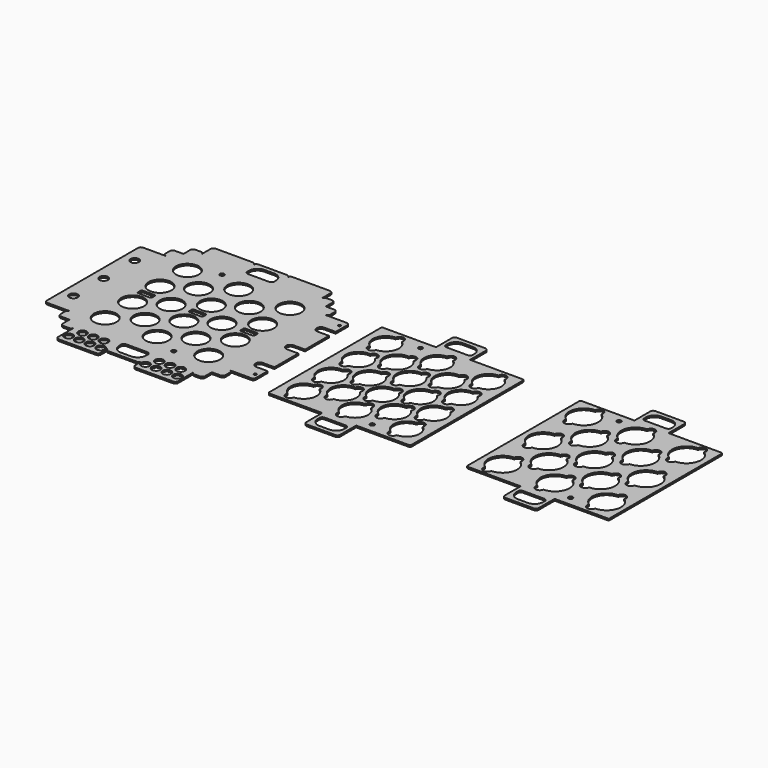
from build123d import *

# Parameters (mm, degrees)
F0_R     = 15
F0_R_2   = 40
F0_R_3   = 7.5
F0_R_4   = 4.25
F1_DEPTH = 6
F2_R     = 7.5
F3_DEPTH = 6
F4_DEPTH = 6


# Not quite as in the source:
# - ends of sketch curves that miss each other by under 0.0002 mm in the source are joined
# - a feature names something its author has since deleted; it is built from what else it names


with BuildPart() as f1:
    # F0 (on Top) → F1 (new body)
    with BuildSketch(Plane.XY):
        with BuildLine():
            Line((-30, 0), (0, 0))
            Line((0, 0), (0, -30))
            ThreePointArc((0, -30), (2.9289321881, -37.0710678119), (10, -40))
            Line((10, -40), (30, -40))
            ThreePointArc((30, -40), (37.0710678119, -37.0710678119), (40, -30))
            Line((40, -30), (40, -70))
            Line((40, -70), (40, -100))
            ThreePointArc((40, -100), (42.9289321881, -107.0710678119), (50, -110))
            Line((50, -110), (181, -110))
            ThreePointArc((181, -110), (188.0710678119, -107.0710678119), (191, -100))
            Line((191, -100), (191, -70))
            ThreePointArc((191, -70), (193.9289321881, -77.0710678119), (201, -80))
            Line((201, -80), (251, -80))
            Line((251, -80), (301, -80))
            ThreePointArc((301, -80), (308.0710678119, -77.0710678119), (311, -70))
            Line((311, -70), (311, -99.9810798484))
            ThreePointArc((311, -99.9810798484), (313.9356373432, -107.0588464633), (321.0189560508, -109.9810618818))
            Line((321.0189560508, -109.9810618818), (452.8887964343, -109.7310882936))
            ThreePointArc((452.8887964343, -109.7310882936), (459.9476069984, -106.795468917), (462.8698403835, -99.7311062602))
            Line((462.8698403835, -99.7311062602), (462.8698403835, -30))
            ThreePointArc((462.8698403835, -30), (465.7987725717, -37.0710678119), (472.8698403835, -40))
            Line((472.8698403835, -40), (492, -40))
            ThreePointArc((492, -40), (499.0710678119, -37.0710678119), (502, -30))
            Line((502, -30), (502, 0))
            Line((502, 0), (532, 0))
            ThreePointArc((532, 0), (539.0710678119, 2.9289321881), (542, 10))
            Line((542, 10), (542, 30))
            ThreePointArc((542, 30), (539.0710678119, 37.0710678119), (532, 40))
            Line((532, 40), (608, 40))
            ThreePointArc((608, 40), (615.0710678119, 42.9289321881), (618, 50))
            Line((618, 50), (618, 101))
            Line((618, 101), (578, 101))
            ThreePointArc((578, 101), (563, 116), (578, 131))
            Line((578, 131), (618, 131))
            Line((618, 131), (618, 236))
            Line((618, 236), (578, 236))
            ThreePointArc((578, 236), (563, 251), (578, 266))
            Line((578, 266), (618, 266))
            Line((618, 266), (618, 371))
            Line((618, 371), (578, 371))
            ThreePointArc((578, 371), (563, 386), (578, 401))
            Line((578, 401), (618, 401))
            Line((618, 401), (618, 452))
            ThreePointArc((618, 452), (615.0710678119, 459.0710678119), (608, 462))
            Line((608, 462), (532, 462))
            ThreePointArc((532, 462), (539.0710678119, 464.9289321881), (542, 472))
            Line((542, 472), (542, 492))
            ThreePointArc((542, 492), (539.0710678119, 499.0710678119), (532, 502))
            Line((532, 502), (502, 502))
            Line((502, 502), (502, 532))
            ThreePointArc((502, 532), (499.0710678119, 539.0710678119), (492, 542))
            Line((492, 542), (472.8698403835, 542))
            ThreePointArc((472.8698403835, 542), (465.7987725717, 539.0710678119), (462.8698403835, 532))
            Line((462.8698403835, 532), (462.8698403835, 572))
            ThreePointArc((462.8698403835, 572), (459.9409081954, 579.0710678119), (452.8698403835, 582))
            Line((452.8698403835, 582), (321, 582))
            ThreePointArc((321, 582), (313.9289321881, 579.0710678119), (311, 572))
            ThreePointArc((311, 572), (308.0710678119, 579.0710678119), (301, 582))
            Line((301, 582), (251, 582))
            Line((251, 582), (201, 582))
            ThreePointArc((201, 582), (193.9289321881, 579.0710678119), (191, 572))
            ThreePointArc((191, 572), (188.0710678119, 579.0710678119), (181, 582))
            Line((181, 582), (50, 582))
            ThreePointArc((50, 582), (42.9289321881, 579.0710678119), (40, 572))
            Line((40, 572), (40, 532))
            ThreePointArc((40, 532), (37.0710678119, 539.0710678119), (30, 542))
            Line((30, 542), (10, 542))
            ThreePointArc((10, 542), (2.9289321881, 539.0710678119), (0, 532))
            Line((0, 532), (0, 502))
            Line((0, 502), (-30, 502))
            ThreePointArc((-30, 502), (-37.0710678119, 499.0710678119), (-40, 492))
            Line((-40, 492), (-40, 472))
            ThreePointArc((-40, 472), (-37.0710678119, 464.9289321881), (-30, 462))
            Line((-30, 462), (-110, 462))
            ThreePointArc((-110, 462), (-117.0710678119, 459.0710678119), (-120, 452))
            Line((-120, 452), (-120, 251))
            Line((-120, 251), (-120, 50))
            ThreePointArc((-120, 50), (-117.0710678119, 42.9289321881), (-110, 40))
            Line((-110, 40), (-30, 40))
            ThreePointArc((-30, 40), (-37.0710678119, 37.0710678119), (-40, 30))
            Line((-40, 30), (-40, 10))
            ThreePointArc((-40, 10), (-37.0710678119, 2.9289321881), (-30, 0))
        make_face()
        with Locations((58.8749991059, -77.75)):
            Circle(F0_R, mode=Mode.SUBTRACT)
        with Locations((96.6249991059, -77.75)):
            Circle(F0_R, mode=Mode.SUBTRACT)
        with Locations((134.3749991059, -77.75)):
            Circle(F0_R, mode=Mode.SUBTRACT)
        with Locations((77.7499991059, -40)):
            Circle(F0_R, mode=Mode.SUBTRACT)
        with Locations((115.4999991059, -40)):
            Circle(F0_R, mode=Mode.SUBTRACT)
        with Locations((153.2499991059, -40)):
            Circle(F0_R, mode=Mode.SUBTRACT)
        with Locations((172.1249991059, -77.75)):
            Circle(F0_R, mode=Mode.SUBTRACT)
        with Locations((-80, 117.4095802605)):
            Circle(F0_R, mode=Mode.SUBTRACT)
        with Locations((70.0655404942, 69.6284726141)):
            Circle(F0_R_2, mode=Mode.SUBTRACT)
        with Locations((162.0928294033, 130.3333938122)):
            Circle(F0_R_2, mode=Mode.SUBTRACT)
        with Locations((70, 190.6667947769)):
            Circle(F0_R_2, mode=Mode.SUBTRACT)
        with Locations((329.8749991059, -77.75)):
            Circle(F0_R, mode=Mode.SUBTRACT)
        with BuildLine():
            Line((298.4369397163, -27.4369397163), (298.4369397163, -35))
            ThreePointArc((298.4369397163, -35), (289.6501431519, -56.2132034356), (268.4369397163, -65))
            Line((268.4369397163, -65), (233.5630602837, -65))
            ThreePointArc((233.5630602837, -65), (212.3498568481, -56.2132034356), (203.5630602837, -35))
            Line((203.5630602837, -35), (203.5630602837, -27.4369397163))
            ThreePointArc((203.5630602837, -27.4369397163), (206.4919924718, -20.3658719045), (213.5630602837, -17.4369397163))
            Line((213.5630602837, -17.4369397163), (288.4369397163, -17.4369397163))
            ThreePointArc((288.4369397163, -17.4369397163), (295.5080075282, -20.3658719045), (298.4369397163, -27.4369397163))
        make_face(mode=Mode.SUBTRACT)
        with Locations((367.6249991059, -77.75)):
            Circle(F0_R, mode=Mode.SUBTRACT)
        with Locations((405.3749991059, -77.75)):
            Circle(F0_R, mode=Mode.SUBTRACT)
        with Locations((348.7499991059, -40)):
            Circle(F0_R, mode=Mode.SUBTRACT)
        with Locations((386.4999991059, -40)):
            Circle(F0_R, mode=Mode.SUBTRACT)
        with Locations((424.2499991059, -40)):
            Circle(F0_R, mode=Mode.SUBTRACT)
        with Locations((341.500023365, 32.5)):
            Circle(F0_R_3, mode=Mode.SUBTRACT)
        with Locations((443.1249991059, -77.75)):
            Circle(F0_R, mode=Mode.SUBTRACT)
        with Locations((250.9999752045, 72.1276074222)):
            Circle(F0_R_2, mode=Mode.SUBTRACT)
        with Locations((432.5207205657, 72.8690030603)):
            Circle(F0_R_2, mode=Mode.SUBTRACT)
        with Locations((341.4999717873, 130.3333938122)):
            Circle(F0_R_2, mode=Mode.SUBTRACT)
        with Locations((250.999969244, 190.6667947769)):
            Circle(F0_R_2, mode=Mode.SUBTRACT)
        with BuildLine():
            ThreePointArc((431.9999940395, 230.6666), (432.2603582464, 230.665752622), (432.520711422, 230.663210524))
            ThreePointArc((432.520711422, 230.663210524), (460.4677713966, 218.7661667645), (471.9999940395, 190.6666))
            ThreePointArc((471.9999940395, 190.6666), (403.7157227921, 162.3823287525), (431.9999940395, 230.6666))
        make_face(mode=Mode.SUBTRACT)
        with Locations((603, 65)):
            Circle(F0_R_4, mode=Mode.SUBTRACT)
        with Locations((-80, 251)):
            Circle(F0_R, mode=Mode.SUBTRACT)
        with Locations((-80, 387.4095802605)):
            Circle(F0_R, mode=Mode.SUBTRACT)
        with BuildLine():
            Line((95, 256), (95, 246))
            ThreePointArc((95, 246), (93.5355339059, 242.4644660941), (90, 241))
            Line((90, 241), (50, 241))
            ThreePointArc((50, 241), (46.4644660941, 242.4644660941), (45, 246))
            Line((45, 246), (45, 256))
            ThreePointArc((45, 256), (46.4644660941, 259.5355339059), (50, 261))
            Line((50, 261), (90, 261))
            ThreePointArc((90, 261), (93.5355339059, 259.5355339059), (95, 256))
        make_face(mode=Mode.SUBTRACT)
        with Locations((70, 311.3332052231)):
            Circle(F0_R_2, mode=Mode.SUBTRACT)
        with Locations((162.1251841753, 245.0216537661)):
            Circle(F0_R_2, mode=Mode.SUBTRACT)
        with Locations((162.1251583099, 365.6882350202)):
            Circle(F0_R_2, mode=Mode.SUBTRACT)
        with Locations((70, 431.9998052231)):
            Circle(F0_R_2, mode=Mode.SUBTRACT)
        with Locations((160.5000174046, 471.9999026115)):
            Circle(F0_R_3, mode=Mode.SUBTRACT)
        with BuildLine():
            ThreePointArc((231.0000407696, 241), (227.4645068636, 242.4644660941), (226.0000407696, 246))
            Line((226.0000407696, 246), (226.0000407696, 256))
            ThreePointArc((226.0000407696, 256), (227.4645068636, 259.5355339059), (231.0000407696, 261))
            Line((231.0000407696, 261), (271.0000407696, 261))
            ThreePointArc((271.0000407696, 261), (274.5355746755, 259.5355339059), (276.0000407696, 256))
            Line((276.0000407696, 256), (276.0000407696, 246))
            ThreePointArc((276.0000407696, 246), (274.5355746755, 242.4644660941), (271.0000407696, 241))
            Line((271.0000407696, 241), (231.0000407696, 241))
        make_face(mode=Mode.SUBTRACT)
        with Locations((250.999969244, 311.3333880901)):
            Circle(F0_R_2, mode=Mode.SUBTRACT)
        with Locations((341.5323265593, 245.0216537661)):
            Circle(F0_R_2, mode=Mode.SUBTRACT)
        with BuildLine():
            Line((457.5207149068, 255.9999994954), (457.5207138976, 245.9999994954))
            ThreePointArc((457.5207138976, 245.9999994954), (456.0562476252, 242.4644659157), (452.5207138976, 241))
            Line((452.5207138976, 241), (412.520711422, 241))
            ThreePointArc((412.520711422, 241), (408.985177516, 242.4644660941), (407.520711422, 246))
            Line((407.520711422, 246), (407.520711422, 256))
            ThreePointArc((407.520711422, 256), (408.985177516, 259.5355339059), (412.520711422, 261))
            Line((412.520711422, 261), (452.5207149068, 261))
            ThreePointArc((452.5207149068, 261), (456.0562489911, 259.5355337275), (457.5207149068, 255.9999994954))
        make_face(mode=Mode.SUBTRACT)
        with BuildLine():
            ThreePointArc((432.5207173824, 271.3365946991), (432.2603642069, 271.3340526011), (432, 271.3332052231))
            ThreePointArc((432, 271.3332052231), (403.7157287525, 339.6174764705), (472, 311.3332052231))
            ThreePointArc((472, 311.3332052231), (460.467777357, 283.2336384586), (432.5207173824, 271.3365946991))
        make_face(mode=Mode.SUBTRACT)
        with Locations((341.5323006939, 365.6882350202)):
            Circle(F0_R_2, mode=Mode.SUBTRACT)
        with Locations((251.0000348091, 432)):
            Circle(F0_R_2, mode=Mode.SUBTRACT)
        with Locations((432.0000112057, 431.9922370985)):
            Circle(F0_R_2, mode=Mode.SUBTRACT)
        with BuildLine():
            Line((288.4369397163, 519.4369397163), (213.5630602837, 519.4369397163))
            ThreePointArc((213.5630602837, 519.4369397163), (206.4919924718, 522.3658719045), (203.5630602837, 529.4369397163))
            Line((203.5630602837, 529.4369397163), (203.5630602837, 537))
            ThreePointArc((203.5630602837, 537), (212.3498568481, 558.2132034356), (233.5630602837, 567))
            Line((233.5630602837, 567), (268.4369397163, 567))
            ThreePointArc((268.4369397163, 567), (289.6501431519, 558.2132034356), (298.4369397163, 537))
            Line((298.4369397163, 537), (298.4369397163, 529.4369397163))
            ThreePointArc((298.4369397163, 529.4369397163), (295.5080075282, 522.3658719045), (288.4369397163, 519.4369397163))
        make_face(mode=Mode.SUBTRACT)
        with Locations((603, 437)):
            Circle(F0_R_4, mode=Mode.SUBTRACT)
    extrude(amount=F1_DEPTH)


with BuildPart() as f3:
    # F2 (on Top) → F3 (new body)
    with BuildSketch(Plane.XY):
        with BuildLine():
            ThreePointArc((700, 5), (701.4644660941, 1.4644660941), (705, 0))
            Line((705, 0), (891.0000348091, 0))
            Line((891.0000348091, 0), (891.0000348091, -70))
            ThreePointArc((891.0000348091, -70), (893.9289669972, -77.0710678119), (901.0000348091, -80))
            Line((901.0000348091, -80), (1001.0000348091, -80))
            ThreePointArc((1001.0000348091, -80), (1008.071102621, -77.0710678119), (1011.0000348091, -70))
            Line((1011.0000348091, -70), (1011.0000348091, 0))
            Line((1011.0000348091, 0), (1197, 0))
            ThreePointArc((1197, 0), (1200.5355339059, 1.4644660941), (1202, 5))
            Line((1202, 5), (1202, 497))
            ThreePointArc((1202, 497), (1200.5355339059, 500.5355339059), (1197, 502))
            Line((1197, 502), (1011.0000348091, 502))
            Line((1011.0000348091, 502), (1011.0000348091, 572))
            ThreePointArc((1011.0000348091, 572), (1008.071102621, 579.0710678119), (1001.0000348091, 582))
            Line((1001.0000348091, 582), (951.0000348091, 582))
            Line((951.0000348091, 582), (901.0000348091, 582))
            ThreePointArc((901.0000348091, 582), (893.9289669972, 579.0710678119), (891.0000348091, 572))
            Line((891.0000348091, 572), (891.0000348091, 502))
            Line((891.0000348091, 502), (705, 502))
            ThreePointArc((705, 502), (701.4644660941, 500.5355339059), (700, 497))
            Line((700, 497), (700, 5))
        make_face()
        with BuildLine():
            ThreePointArc((903.5630950928, -27.4369397163), (906.4920272809, -20.3658719045), (913.5630950928, -17.4369397163))
            Line((913.5630950928, -17.4369397163), (988.4369745255, -17.4369397163))
            ThreePointArc((988.4369745255, -17.4369397163), (995.5080423373, -20.3658719045), (998.4369745255, -27.4369397163))
            Line((998.4369745255, -27.4369397163), (998.4369745255, -35))
            ThreePointArc((998.4369745255, -35), (989.650177961, -56.2132034356), (968.4369745255, -65))
            Line((968.4369745255, -65), (933.5630950928, -65))
            ThreePointArc((933.5630950928, -65), (912.3498916572, -56.2132034356), (903.5630950928, -35))
            Line((903.5630950928, -35), (903.5630950928, -27.4369397163))
        make_face(mode=Mode.SUBTRACT)
        with BuildLine():
            ThreePointArc((743.4629290669, 32.1011350421), (725.9747079734, 82.7432920036), (768.2980336481, 115.5945026749))
            ThreePointArc((768.2980336481, 115.5945026749), (787.4569314238, 128.0967505221), (796.6681519216, 107.1558101861))
            ThreePointArc((796.6681519216, 107.1558101861), (814.1563730151, 56.5136532246), (771.8330473404, 23.6624425533))
            ThreePointArc((771.8330473404, 23.6624425533), (752.6741495647, 11.160194706), (743.4629290669, 32.1011350421))
        make_face(mode=Mode.SUBTRACT)
        with BuildLine():
            ThreePointArc((924.3973637771, 32.472676362), (906.9091426836, 83.1148333236), (949.2324683583, 115.9660439948))
            ThreePointArc((949.2324683583, 115.9660439948), (968.391366134, 128.4682918421), (977.6025866319, 107.5273515061))
            ThreePointArc((977.6025866319, 107.5273515061), (995.0908077253, 56.8851945445), (952.7674820507, 24.0339838733))
            ThreePointArc((952.7674820507, 24.0339838733), (933.6085842749, 11.531736026), (924.3973637771, 32.472676362))
        make_face(mode=Mode.SUBTRACT)
        with Locations((1041.5, 32.5)):
            Circle(F2_R, mode=Mode.SUBTRACT)
        with BuildLine():
            ThreePointArc((1105.8087297084, 33.2918495689), (1088.4298880449, 83.8562289617), (1130.619107199, 116.7020869672))
            ThreePointArc((1130.619107199, 116.7020869672), (1149.7414459012, 129.2601810812), (1159.0137260989, 108.346205248))
            ThreePointArc((1159.0137260989, 108.346205248), (1176.6115530866, 57.6265901827), (1134.1541058449, 24.7704181479))
            ThreePointArc((1134.1541058449, 24.7704181479), (1114.9588120925, 12.3241229973), (1105.8087297084, 33.2918495689))
        make_face(mode=Mode.SUBTRACT)
        with BuildLine():
            ThreePointArc((835.4902179759, 92.8060562402), (819.0847524845, 146.6522577354), (867.080685302, 176.0621735196))
            ThreePointArc((867.080685302, 176.0621735196), (887.8649251028, 185.6217206385), (893.907820072, 163.5569753282))
            ThreePointArc((893.907820072, 163.5569753282), (905.1009063221, 114.0145298889), (863.8603362495, 84.3673637514))
            ThreePointArc((863.8603362495, 84.3673637514), (844.7014384737, 71.8651159041), (835.4902179759, 92.8060562402))
        make_face(mode=Mode.SUBTRACT)
        with BuildLine():
            ThreePointArc((743.3973885726, 153.1394572049), (726.9919230812, 206.9856587001), (774.9878558987, 236.3955744844))
            ThreePointArc((774.9878558987, 236.3955744844), (795.7720956995, 245.9551216032), (801.8149906687, 223.8903762929))
            ThreePointArc((801.8149906687, 223.8903762929), (813.0080769188, 174.3479308537), (771.7675068462, 144.7007647161))
            ThreePointArc((771.7675068462, 144.7007647161), (752.6086090704, 132.1985168689), (743.3973885726, 153.1394572049))
        make_face(mode=Mode.SUBTRACT)
        with BuildLine():
            ThreePointArc((924.3973637771, 153.1394572049), (907.9918982856, 206.9856587001), (955.9878311031, 236.3955744844))
            ThreePointArc((955.9878311031, 236.3955744844), (976.772070904, 245.9551216032), (982.8149658732, 223.8903762929))
            ThreePointArc((982.8149658732, 223.8903762929), (994.0080521233, 174.3479308537), (952.7674820507, 144.7007647161))
            ThreePointArc((952.7674820507, 144.7007647161), (933.6085842749, 132.1985168689), (924.3973637771, 153.1394572049))
        make_face(mode=Mode.SUBTRACT)
        with BuildLine():
            ThreePointArc((835.5225727479, 207.4943161941), (819.1171072565, 261.3405176894), (867.1130400739, 290.7504334736))
            ThreePointArc((867.1130400739, 290.7504334736), (887.8972798748, 300.3099805924), (893.940174844, 278.2452352821))
            ThreePointArc((893.940174844, 278.2452352821), (905.1332610941, 228.7027898429), (863.8926910215, 199.0556237053))
            ThreePointArc((863.8926910215, 199.0556237053), (844.7337932457, 186.5533758581), (835.5225727479, 207.4943161941))
        make_face(mode=Mode.SUBTRACT)
        with BuildLine():
            ThreePointArc((1014.8973603599, 92.8060562402), (998.4918948685, 146.6522577354), (1046.487827686, 176.0621735196))
            ThreePointArc((1046.487827686, 176.0621735196), (1067.2720674868, 185.6217206385), (1073.314962456, 163.5569753282))
            ThreePointArc((1073.314962456, 163.5569753282), (1084.5080487061, 114.0145298889), (1043.2674786335, 84.3673637514))
            ThreePointArc((1043.2674786335, 84.3673637514), (1024.1085808577, 71.8651159041), (1014.8973603599, 92.8060562402))
        make_face(mode=Mode.SUBTRACT)
        with BuildLine():
            ThreePointArc((1105.3973885726, 153.1394572049), (1088.9919230812, 206.9856587001), (1136.9878558987, 236.3955744844))
            ThreePointArc((1136.9878558987, 236.3955744844), (1157.7720956995, 245.9551216032), (1163.8149906687, 223.8903762929))
            ThreePointArc((1163.8149906687, 223.8903762929), (1175.0080769188, 174.3479308537), (1133.7675068462, 144.7007647161))
            ThreePointArc((1133.7675068462, 144.7007647161), (1114.6086090704, 132.1985168689), (1105.3973885726, 153.1394572049))
        make_face(mode=Mode.SUBTRACT)
        with BuildLine():
            ThreePointArc((1014.9297151319, 207.4943161941), (998.5242496405, 261.3405176894), (1046.5201824579, 290.7504334736))
            ThreePointArc((1046.5201824579, 290.7504334736), (1067.3044222588, 300.3099805924), (1073.347317228, 278.2452352821))
            ThreePointArc((1073.347317228, 278.2452352821), (1084.5404034781, 228.7027898429), (1043.2998334055, 199.0556237053))
            ThreePointArc((1043.2998334055, 199.0556237053), (1024.1409356297, 186.5533758581), (1014.9297151319, 207.4943161941))
        make_face(mode=Mode.SUBTRACT)
        with BuildLine():
            ThreePointArc((743.3973906407, 273.8060506991), (726.9919251493, 327.6522521943), (774.9878579668, 357.0621679785))
            ThreePointArc((774.9878579668, 357.0621679785), (795.7720977677, 366.6217150974), (801.8149927368, 344.5569697871))
            ThreePointArc((801.8149927368, 344.5569697871), (813.0080789869, 295.0145243478), (771.7675089143, 265.3673582103))
            ThreePointArc((771.7675089143, 265.3673582103), (752.6086111386, 252.865110363), (743.3973906407, 273.8060506991))
        make_face(mode=Mode.SUBTRACT)
        with BuildLine():
            ThreePointArc((924.3973637771, 273.8060505181), (907.9918982856, 327.6522520134), (955.9878311031, 357.0621677976))
            ThreePointArc((955.9878311031, 357.0621677976), (976.772070904, 366.6217149165), (982.8149658732, 344.5569696061))
            ThreePointArc((982.8149658732, 344.5569696061), (994.0080521233, 295.0145241669), (952.7674820507, 265.3673580294))
            ThreePointArc((952.7674820507, 265.3673580294), (933.6085842749, 252.8651101821), (924.3973637771, 273.8060505181))
        make_face(mode=Mode.SUBTRACT)
        with BuildLine():
            ThreePointArc((835.5225468826, 328.1608974482), (819.1170813911, 382.0070989434), (867.1130142086, 411.4170147276))
            ThreePointArc((867.1130142086, 411.4170147276), (887.8972540095, 420.9765618465), (893.9401489786, 398.9118165362))
            ThreePointArc((893.9401489786, 398.9118165362), (905.1332352288, 349.3693710969), (863.8926651561, 319.7222049594))
            ThreePointArc((863.8926651561, 319.7222049594), (844.7337673804, 307.2199571121), (835.5225468826, 328.1608974482))
        make_face(mode=Mode.SUBTRACT)
        with BuildLine():
            ThreePointArc((1105.3973906407, 273.8060506991), (1088.9919251493, 327.6522521943), (1136.9878579668, 357.0621679785))
            ThreePointArc((1136.9878579668, 357.0621679785), (1157.7720977677, 366.6217150974), (1163.8149927368, 344.5569697871))
            ThreePointArc((1163.8149927368, 344.5569697871), (1175.0080789869, 295.0145243478), (1133.7675089143, 265.3673582103))
            ThreePointArc((1133.7675089143, 265.3673582103), (1114.6086111386, 252.865110363), (1105.3973906407, 273.8060506991))
        make_face(mode=Mode.SUBTRACT)
        with BuildLine():
            ThreePointArc((1014.9296892666, 328.1608974482), (998.5242237751, 382.0070989434), (1046.5201565926, 411.4170147276))
            ThreePointArc((1046.5201565926, 411.4170147276), (1067.3043963935, 420.9765618465), (1073.3472913626, 398.9118165362))
            ThreePointArc((1073.3472913626, 398.9118165362), (1084.5403776128, 349.3693710969), (1043.2998075401, 319.7222049594))
            ThreePointArc((1043.2998075401, 319.7222049594), (1024.1409097644, 307.2199571121), (1014.9296892666, 328.1608974482))
        make_face(mode=Mode.SUBTRACT)
        with BuildLine():
            ThreePointArc((743.3973694991, 394.472662428), (725.9091484057, 445.1148193895), (768.2324740803, 477.9660300608))
            ThreePointArc((768.2324740803, 477.9660300608), (787.3913718561, 490.4682779081), (796.6025923539, 469.527337572))
            ThreePointArc((796.6025923539, 469.527337572), (814.0908134473, 418.8851806105), (771.7674877727, 386.0339699392))
            ThreePointArc((771.7674877727, 386.0339699392), (752.6085899969, 373.5317220919), (743.3973694991, 394.472662428))
        make_face(mode=Mode.SUBTRACT)
        with BuildLine():
            ThreePointArc((924.3974233817, 394.472662428), (906.9092022883, 445.1148193895), (949.2325279629, 477.9660300608))
            ThreePointArc((949.2325279629, 477.9660300608), (968.3914257387, 490.4682779081), (977.6026462365, 469.527337572))
            ThreePointArc((977.6026462365, 469.527337572), (995.0908673299, 418.8851806105), (952.7675416553, 386.0339699392))
            ThreePointArc((952.7675416553, 386.0339699392), (933.6086438795, 373.5317220919), (924.3974233817, 394.472662428))
        make_face(mode=Mode.SUBTRACT)
        with Locations((860.5, 471.5)):
            Circle(F2_R, mode=Mode.SUBTRACT)
        with BuildLine():
            Line((988.4369745255, 519.4368882179), (913.5630950928, 519.4368882179))
            ThreePointArc((913.5630950928, 519.4368882179), (906.4920272809, 522.3658204061), (903.5630950928, 529.4368882179))
            Line((903.5630950928, 529.4368882179), (903.5630950928, 536.9999485016))
            ThreePointArc((903.5630950928, 536.9999485016), (912.3498916572, 558.2131519372), (933.5630950928, 566.9999485016))
            Line((933.5630950928, 566.9999485016), (968.4369745255, 566.9999485016))
            ThreePointArc((968.4369745255, 566.9999485016), (989.650177961, 558.2131519372), (998.4369745255, 536.9999485016))
            Line((998.4369745255, 536.9999485016), (998.4369745255, 529.4368882179))
            ThreePointArc((998.4369745255, 529.4368882179), (995.5080423373, 522.3658204061), (988.4369745255, 519.4368882179))
        make_face(mode=Mode.SUBTRACT)
        with BuildLine():
            ThreePointArc((1105.3973885726, 394.4726736337), (1087.9091674792, 445.1148305952), (1130.2324931538, 477.9660412665))
            ThreePointArc((1130.2324931538, 477.9660412665), (1149.3913909296, 490.4682891137), (1158.6026114274, 469.5273487777))
            ThreePointArc((1158.6026114274, 469.5273487777), (1176.0908325208, 418.8851918162), (1133.7675068462, 386.0339811449))
            ThreePointArc((1133.7675068462, 386.0339811449), (1114.6086090704, 373.5317332976), (1105.3973885726, 394.4726736337))
        make_face(mode=Mode.SUBTRACT)
    extrude(amount=F3_DEPTH)


with BuildPart() as f4:
    # F2 (on Top) → F4 (new body)
    with BuildSketch(Plane.XY):
        with BuildLine():
            Line((1710.9677224929, 0), (1901.9999761581, 0))
            Line((1901.9999761581, 0), (1901.9999761581, 497))
            ThreePointArc((1901.9999761581, 497), (1900.5355339059, 500.5355339059), (1897, 502))
            Line((1897, 502), (1710.9677224929, 502))
            Line((1710.9677224929, 502), (1710.9677224929, 572))
            ThreePointArc((1710.9677224929, 572), (1708.0387903048, 579.0710678119), (1700.9677224929, 582))
            Line((1700.9677224929, 582), (1650.9677224929, 582))
            Line((1650.9677224929, 582), (1600.9677224929, 582))
            ThreePointArc((1600.9677224929, 582), (1593.896654681, 579.0710678119), (1590.9677224929, 572))
            Line((1590.9677224929, 572), (1590.9677224929, 502))
            Line((1590.9677224929, 502), (1404.9999761581, 502))
            ThreePointArc((1404.9999761581, 502), (1401.4644422522, 500.5355339059), (1399.9999761581, 497))
            Line((1399.9999761581, 497), (1399.9999761581, 5))
            ThreePointArc((1399.9999761581, 5), (1401.4644422522, 1.4644660941), (1404.9999761581, 0))
            Line((1404.9999761581, 0), (1590.9999761581, 0))
            Line((1590.9999761581, 0), (1590.9999761581, -70))
            ThreePointArc((1590.9999761581, -70), (1593.9289083463, -77.0710678119), (1600.9999761581, -80))
            Line((1600.9999761581, -80), (1650.9677224929, -80))
            Line((1650.9677224929, -80), (1650.9999761581, -80))
            Line((1650.9999761581, -80), (1700.9677224929, -80))
            ThreePointArc((1700.9677224929, -80), (1708.0387903048, -77.0710678119), (1710.9677224929, -70))
            Line((1710.9677224929, -70), (1710.9677224929, 0))
        make_face()
        with BuildLine():
            ThreePointArc((1442.3992554122, 29.2403812138), (1421.6485069343, 86.3196329847), (1470.2221267258, 122.7783494389))
            ThreePointArc((1470.2221267258, 122.7783494389), (1489.3487360272, 135.0400494523), (1498.6643870896, 114.3181982833))
            ThreePointArc((1498.6643870896, 114.3181982833), (1519.4151355675, 57.2389465123), (1470.8415157761, 20.7802300582))
            ThreePointArc((1470.8415157761, 20.7802300582), (1451.7149064747, 8.5185300447), (1442.3992554122, 29.2403812138))
        make_face(mode=Mode.SUBTRACT)
        with BuildLine():
            ThreePointArc((1603.5307827765, -27.4369397163), (1606.4597149647, -20.3658719045), (1613.5307827765, -17.4369397163))
            Line((1613.5307827765, -17.4369397163), (1688.4046622092, -17.4369397163))
            ThreePointArc((1688.4046622092, -17.4369397163), (1695.4757300211, -20.3658719045), (1698.4046622092, -27.4369397163))
            Line((1698.4046622092, -27.4369397163), (1698.4046622092, -35))
            ThreePointArc((1698.4046622092, -35), (1689.6178656448, -56.2132034356), (1668.4046622092, -65))
            Line((1668.4046622092, -65), (1633.5307827765, -65))
            ThreePointArc((1633.5307827765, -65), (1612.3175793409, -56.2132034356), (1603.5307827765, -35))
            Line((1603.5307827765, -35), (1603.5307827765, -27.4369397163))
        make_face(mode=Mode.SUBTRACT)
        with Locations((1741.5, 32.5)):
            Circle(F2_R, mode=Mode.SUBTRACT)
        with BuildLine():
            ThreePointArc((1624.2929093706, 32.253587195), (1603.5421608927, 89.332838966), (1652.1157806842, 125.7915554202))
            ThreePointArc((1652.1157806842, 125.7915554202), (1671.2423899856, 138.0532554336), (1680.558041048, 117.3314042646))
            ThreePointArc((1680.558041048, 117.3314042646), (1701.3087895259, 60.2521524936), (1652.7351697344, 23.7934360394))
            ThreePointArc((1652.7351697344, 23.7934360394), (1633.608560433, 11.531736026), (1624.2929093706, 32.253587195))
        make_face(mode=Mode.SUBTRACT)
        with BuildLine():
            ThreePointArc((1805.703636515, 33.0730660291), (1785.0768831018, 90.0700549867), (1833.5017054112, 126.5276507782))
            ThreePointArc((1833.5017054112, 126.5276507782), (1852.5924576174, 138.845103875), (1861.9685287038, 118.1505209709))
            ThreePointArc((1861.9685287038, 118.1505209709), (1882.843511735, 60.9893685143), (1834.1210918251, 24.5299655453))
            ThreePointArc((1834.1210918251, 24.5299655453), (1814.9587882506, 12.3241229973), (1805.703636515, 33.0730660291))
        make_face(mode=Mode.SUBTRACT)
        with BuildLine():
            ThreePointArc((1532.4238928446, 121.0180695717), (1511.6731443667, 178.0973213427), (1560.2467641581, 214.5560377969))
            ThreePointArc((1560.2467641581, 214.5560377969), (1579.3733734595, 226.8177378103), (1588.689024522, 206.0958866413))
            ThreePointArc((1588.689024522, 206.0958866413), (1609.4397729999, 149.0166348703), (1560.8661532084, 112.5579184161))
            ThreePointArc((1560.8661532084, 112.5579184161), (1541.739543907, 100.2962184027), (1532.4238928446, 121.0180695717))
        make_face(mode=Mode.SUBTRACT)
        with BuildLine():
            ThreePointArc((1714.0542059875, 121.0180695717), (1693.3034575096, 178.0973213427), (1741.8770773011, 214.5560377969))
            ThreePointArc((1741.8770773011, 214.5560377969), (1761.0036866025, 226.8177378103), (1770.3193376649, 206.0958866413))
            ThreePointArc((1770.3193376649, 206.0958866413), (1791.0700861428, 149.0166348703), (1742.4964663513, 112.5579184161))
            ThreePointArc((1742.4964663513, 112.5579184161), (1723.3698570499, 100.2962184027), (1714.0542059875, 121.0180695717))
        make_face(mode=Mode.SUBTRACT)
        with BuildLine():
            ThreePointArc((1441.9001440872, 208.482744879), (1421.1493956093, 265.56199665), (1469.7230154008, 302.0207131041))
            ThreePointArc((1469.7230154008, 302.0207131041), (1488.8496247022, 314.2824131176), (1498.1652757646, 293.5605619486))
            ThreePointArc((1498.1652757646, 293.5605619486), (1518.9160242425, 236.4813101776), (1470.3424044511, 200.0225937234))
            ThreePointArc((1470.3424044511, 200.0225937234), (1451.2157951497, 187.76089371), (1441.9001440872, 208.482744879))
        make_face(mode=Mode.SUBTRACT)
        with BuildLine():
            ThreePointArc((1532.6770740925, 299.2652680342), (1511.9263256146, 356.3445198052), (1560.499945406, 392.8032362593))
            ThreePointArc((1560.499945406, 392.8032362593), (1579.6265547074, 405.0649362728), (1588.9422057699, 384.3430851038))
            ThreePointArc((1588.9422057699, 384.3430851038), (1609.6929542478, 327.2638333328), (1561.1193344563, 290.8051168786))
            ThreePointArc((1561.1193344563, 290.8051168786), (1541.9927251549, 278.5434168652), (1532.6770740925, 299.2652680342))
        make_face(mode=Mode.SUBTRACT)
        with BuildLine():
            ThreePointArc((1622.8673135218, 208.482744879), (1602.1165650439, 265.56199665), (1650.6901848353, 302.0207131041))
            ThreePointArc((1650.6901848353, 302.0207131041), (1669.8167941367, 314.2824131176), (1679.1324451992, 293.5605619486))
            ThreePointArc((1679.1324451992, 293.5605619486), (1699.8831936771, 236.4813101776), (1651.3095738856, 200.0225937234))
            ThreePointArc((1651.3095738856, 200.0225937234), (1632.1829645842, 187.76089371), (1622.8673135218, 208.482744879))
        make_face(mode=Mode.SUBTRACT)
        with BuildLine():
            ThreePointArc((1804.6361128265, 208.482744879), (1783.8853643486, 265.56199665), (1832.45898414, 302.0207131041))
            ThreePointArc((1832.45898414, 302.0207131041), (1851.5855934414, 314.2824131176), (1860.9012445039, 293.5605619486))
            ThreePointArc((1860.9012445039, 293.5605619486), (1881.6519929817, 236.4813101776), (1833.0783731903, 200.0225937234))
            ThreePointArc((1833.0783731903, 200.0225937234), (1813.9517638889, 187.76089371), (1804.6361128265, 208.482744879))
        make_face(mode=Mode.SUBTRACT)
        with BuildLine():
            ThreePointArc((1713.6285225326, 299.0945852208), (1692.8777740547, 356.1738369918), (1741.4513938461, 392.632553446))
            ThreePointArc((1741.4513938461, 392.632553446), (1760.5780031475, 404.8942534594), (1769.89365421, 384.1724022904))
            ThreePointArc((1769.89365421, 384.1724022904), (1790.6444026879, 327.0931505194), (1742.0707828964, 290.6344340652))
            ThreePointArc((1742.0707828964, 290.6344340652), (1722.944173595, 278.3727340518), (1713.6285225326, 299.0945852208))
        make_face(mode=Mode.SUBTRACT)
        with BuildLine():
            ThreePointArc((1440.1653925353, 389.4610914652), (1419.4146440574, 446.5403432362), (1467.9882638489, 482.9990596904))
            ThreePointArc((1467.9882638489, 482.9990596904), (1487.1148731503, 495.2607597038), (1496.4305242127, 474.5389085348))
            ThreePointArc((1496.4305242127, 474.5389085348), (1517.1812726906, 417.4596567638), (1468.6076528992, 381.0009403096))
            ThreePointArc((1468.6076528992, 381.0009403096), (1449.4810435978, 368.7392402962), (1440.1653925353, 389.4610914652))
        make_face(mode=Mode.SUBTRACT)
        with Locations((1560.4999761581, 471.9999)):
            Circle(F2_R, mode=Mode.SUBTRACT)
        with BuildLine():
            ThreePointArc((1622.8673378402, 389.4610914652), (1602.1165893623, 446.5403432362), (1650.6902091538, 482.9990596904))
            ThreePointArc((1650.6902091538, 482.9990596904), (1669.8168184552, 495.2607597038), (1679.1324695176, 474.5389085348))
            ThreePointArc((1679.1324695176, 474.5389085348), (1699.8832179955, 417.4596567638), (1651.309598204, 381.0009403096))
            ThreePointArc((1651.309598204, 381.0009403096), (1632.1829889026, 368.7392402962), (1622.8673378402, 389.4610914652))
        make_face(mode=Mode.SUBTRACT)
        with BuildLine():
            ThreePointArc((1802.4865309173, 389.4610914652), (1781.7357824394, 446.5403432362), (1830.3094022308, 482.9990596904))
            ThreePointArc((1830.3094022308, 482.9990596904), (1849.4360115322, 495.2607597038), (1858.7516625947, 474.5389085348))
            ThreePointArc((1858.7516625947, 474.5389085348), (1879.5024110726, 417.4596567638), (1830.9287912811, 381.0009403096))
            ThreePointArc((1830.9287912811, 381.0009403096), (1811.8021819797, 368.7392402962), (1802.4865309173, 389.4610914652))
        make_face(mode=Mode.SUBTRACT)
        with BuildLine():
            Line((1688.4046622092, 519.4368882179), (1613.5307827765, 519.4368882179))
            ThreePointArc((1613.5307827765, 519.4368882179), (1606.4597149647, 522.3658204061), (1603.5307827765, 529.4368882179))
            Line((1603.5307827765, 529.4368882179), (1603.5307827765, 536.9999485016))
            ThreePointArc((1603.5307827765, 536.9999485016), (1612.3175793409, 558.2131519372), (1633.5307827765, 566.9999485016))
            Line((1633.5307827765, 566.9999485016), (1668.4046622092, 566.9999485016))
            ThreePointArc((1668.4046622092, 566.9999485016), (1689.6178656448, 558.2131519372), (1698.4046622092, 536.9999485016))
            Line((1698.4046622092, 536.9999485016), (1698.4046622092, 529.4368882179))
            ThreePointArc((1698.4046622092, 529.4368882179), (1695.4757300211, 522.3658204061), (1688.4046622092, 519.4368882179))
        make_face(mode=Mode.SUBTRACT)
    extrude(amount=F4_DEPTH)


solid = Compound([f1.part, f3.part, f4.part])
